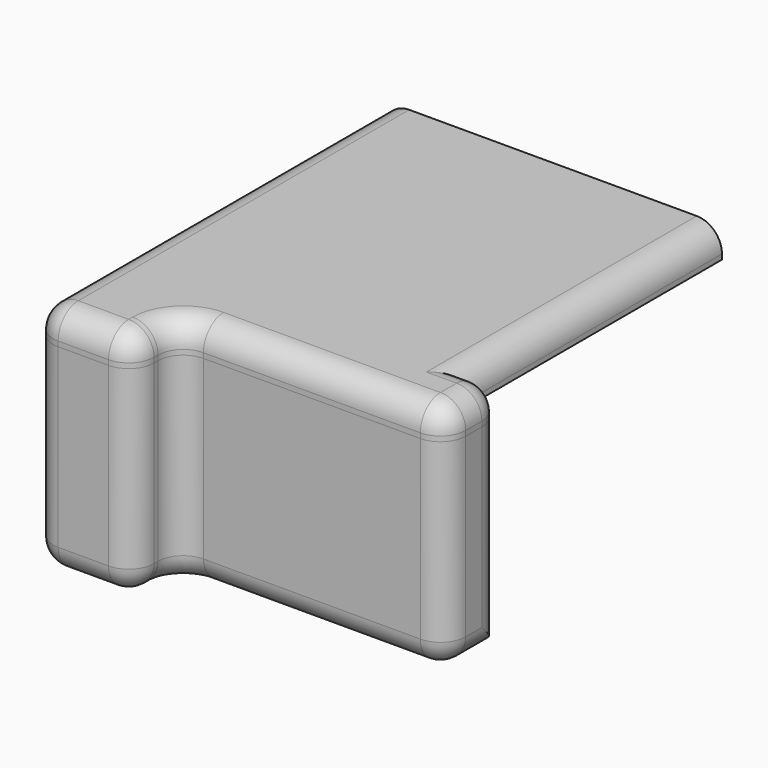
from build123d import *

# Parameters (mm, degrees)
F0_W     = 23.5
F0_H     = 3
F1_DEPTH = 3
F2_DEPTH = 20
F3_R     = 2.5
F3_2_R   = 2.5


with BuildPart() as f1:
    # F0 (on Top) → F1 (new body)
    with BuildSketch(Plane.XY):
        Polygon((-14.4662116915, 31.8095687255), (-14.4662116915, -8.6904312745), (-7.4662116915, -8.6904312745), (-7.4662116915, -3.1904312745), (-4.4662116915, -3.1904312745), (19.0337883085, -3.1904312745), (19.0337883085, 0.8095687255), (19.0337883085, 31.8095687255), align=None)
        Polygon((-7.4662116915, -8.6904312745), (-14.4662116915, -8.6904312745), (-14.4662116915, -11.6904312745), (-7.4662116915, -11.6904312745), (-4.4662116915, -11.6904312745), (-4.4662116915, -6.1904312745), (-4.4662116915, -3.1904312745), (-7.4662116915, -3.1904312745), align=None)
        with Locations((7.2837883085, -4.6904312745)):
            Rectangle(F0_W, F0_H)
        Polygon((22.0337883085, 0.8095687255), (19.0337883085, 0.8095687255), (19.0337883085, -3.1904312745), (19.0337883085, -6.1904312745), (22.0337883085, -6.1904312745), (22.0337883085, -3.1904312745), align=None)
    extrude(amount=F1_DEPTH)

    # F3
    f3_edges = [f1.edges().sort_by_distance(p)[0] for p in [
        (-9.466212, -11.690431, 3),
        (-4.466212, -8.940431, 3),
        (8.783788, -6.190431, 3),
        (22.033788, -2.690431, 3),
        (22.033788, -6.190431, 1.5),
        (-4.466212, -11.690431, 1.5),
        (-4.466212, -6.190431, 1.5),
        (-14.466212, -11.690431, 1.5),
        (-14.466212, 10.059569, 3),
        (20.533788, 0.809569, 3),
        (22.033788, 0.809569, 1.5),
        (19.033788, 16.309569, 3),
    ]]
    fillet(f3_edges, radius=F3_R)


with BuildPart() as f2:
    # F0 (on Top) → F2 (new body)
    with BuildSketch(Plane.XY):
        Polygon((-7.4662116915, -8.6904312745), (-14.4662116915, -8.6904312745), (-14.4662116915, -11.6904312745), (-7.4662116915, -11.6904312745), (-4.4662116915, -11.6904312745), (-4.4662116915, -6.1904312745), (-4.4662116915, -3.1904312745), (-7.4662116915, -3.1904312745), align=None)
        with Locations((7.2837883085, -4.6904312745)):
            Rectangle(F0_W, F0_H)
        Polygon((22.0337883085, 0.8095687255), (19.0337883085, 0.8095687255), (19.0337883085, -3.1904312745), (19.0337883085, -6.1904312745), (22.0337883085, -6.1904312745), (22.0337883085, -3.1904312745), align=None)
    extrude(amount=-F2_DEPTH)

    # F3#2
    f3_2_edges = [f2.edges().sort_by_distance(p)[0] for p in [
        (22.033788, -6.190431, -10),
        (-4.466212, -11.690431, -10),
        (-4.466212, -6.190431, -10),
        (-14.466212, -11.690431, -10),
        (-9.466212, -11.690431, -20),
        (-4.466212, -8.940431, -20),
        (22.033788, -2.690431, -20),
        (-14.466212, -10.190431, -20),
        (22.033788, 0.809569, -10),
        (8.783788, -6.190431, -20),
    ]]
    fillet(f3_2_edges, radius=F3_2_R)


solid = Compound([f1.part, f2.part])
